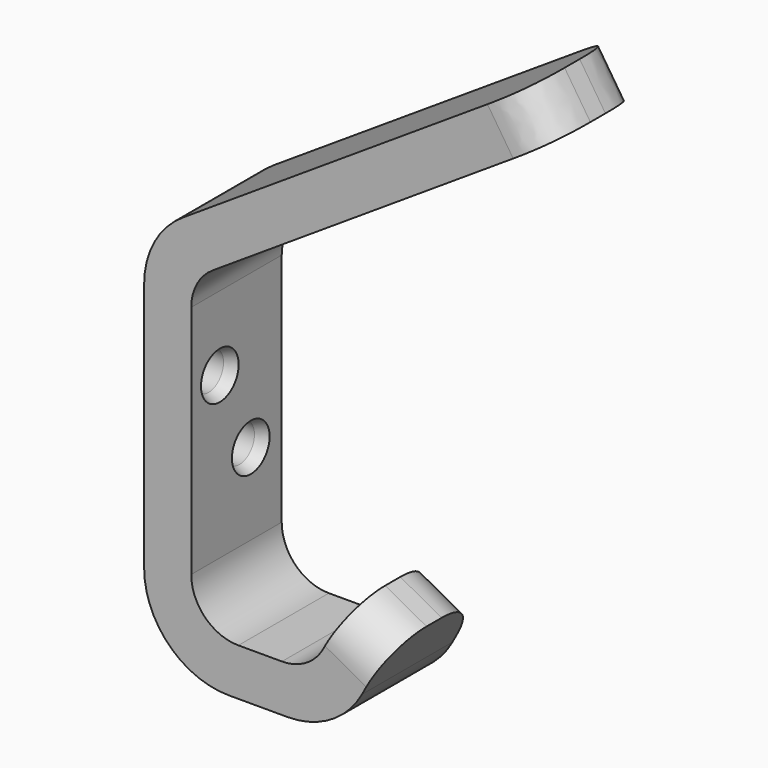
from build123d import *

# Parameters (mm, degrees)
F1_DEPTH        = 12
F2_R            = 9
F3_R            = 5
F4_R            = 9
F5_R            = 5
F6_R            = 5
F7_R            = 5
F8_T1_DEPTH     = 30
F10_R           = 5
F11_R           = 9
F13_D           = 4
F13_CSINK_D     = 5
F13_CSINK_ANGLE = 45
F14_D           = 4
F14_CSINK_D     = 5
F14_CSINK_ANGLE = 45


# Not quite as in the source:
# - a fillet or chamfer that OpenCascade refuses, or shapes differently, is made with other operations: its cross-section is extruded or revolved along the edge and cut away or added


with BuildPart() as f1:
    # F0 (on Front) → F1 (new body)
    with BuildSketch(Plane.XZ):
        Polygon((0, 40.3702630328), (0, 0), (20.5587926316, 0), (25.9716099992, 9.9235005083), (21.5821319316, 12.3177607896), (17.5906268513, 5), (5, 5), (5, 37.6631405767), (43.3543724833, 62.7000143926), (40.621260608, 66.8869105553), align=None)
    extrude(amount=F1_DEPTH)

    # F2
    f2_edges = [f1.edges().sort_by_distance(p)[0] for p in [
        (20.558793, -6, 0),
    ]]
    fillet(f2_edges, radius=F2_R)

    # F3
    f3_edges = [f1.edges().sort_by_distance(p)[0] for p in [
        (17.590627, -6, 5),
    ]]
    fillet(f3_edges, radius=F3_R)

    # F4
    f4_edges = [f1.edges().sort_by_distance(p)[0] for p in [
        (0, -6, 40.370263),
    ]]
    fillet(f4_edges, radius=F4_R)

    # F5
    f5_edges = [f1.edges().sort_by_distance(p)[0] for p in [
        (5, -6, 37.663141),
    ]]
    fillet(f5_edges, radius=F5_R)

    # F6
    f6_edges = [f1.edges().sort_by_distance(p)[0] for p in [
        (23.776871, -12, 11.120631),
    ]]
    fillet(f6_edges, radius=F6_R)

    # F7
    f7_edges = [f1.edges().sort_by_distance(p)[0] for p in [
        (23.776871, 0, 11.120631),
    ]]
    fillet(f7_edges, radius=F7_R)

    # F8: fillet of radius 5 on 2 edges, made by hand

    # F8_s2 → F8_t1 (cut)
    with BuildSketch(Plane(origin=(-8.9127980143, 0, 13.6536525057), x_dir=(0, 1, 0), z_dir=(-0.5466223751, 0, 0.8373792325))):
        with BuildLine():
            add(Edge.make_bspline(
                [(-12, -65.577281941), (-12, -70.577281941), (-7, -70.577281941)],
                knots=[0, 0, 0, 1, 1, 1], degree=2, weights=[1, 1, 1]))
            Line((-7, -70.577281941), (-12, -70.577281941))
            Line((-12, -70.577281941), (-12, -65.577281941))
        make_face()
        with BuildLine():
            add(Edge.make_bspline(
                [(0, -65.577281941), (0, -70.577281941), (-5, -70.577281941)],
                knots=[0, 0, 0, 1, 1, 1], degree=2, weights=[1, 1, 1]))
            Line((-5, -70.577281941), (0, -70.577281941))
            Line((0, -70.577281941), (0, -65.577281941))
        make_face()
    extrude(amount=F8_T1_DEPTH, mode=Mode.SUBTRACT)

    # F10
    f10_edges = [f1.edges().sort_by_distance(p)[0] for p in [
        (5, -6, 5),
    ]]
    fillet(f10_edges, radius=F10_R)

    # F11
    f11_edges = [f1.edges().sort_by_distance(p)[0] for p in [
        (0, -6, 0),
    ]]
    fillet(f11_edges, radius=F11_R)

    # F13 (through all)
    with Locations(Plane.YZ.offset(5)):
        with Locations((-8.210901171, 27.0586498082)):
            CounterSinkHole(F13_D / 2, F13_CSINK_D / 2, counter_sink_angle=F13_CSINK_ANGLE)

    # F14 (through all)
    with Locations(Plane.YZ.offset(5)):
        with Locations((-4.1054510511, 18.6611376703)):
            CounterSinkHole(F14_D / 2, F14_CSINK_D / 2, counter_sink_angle=F14_CSINK_ANGLE)


solid = f1.part
